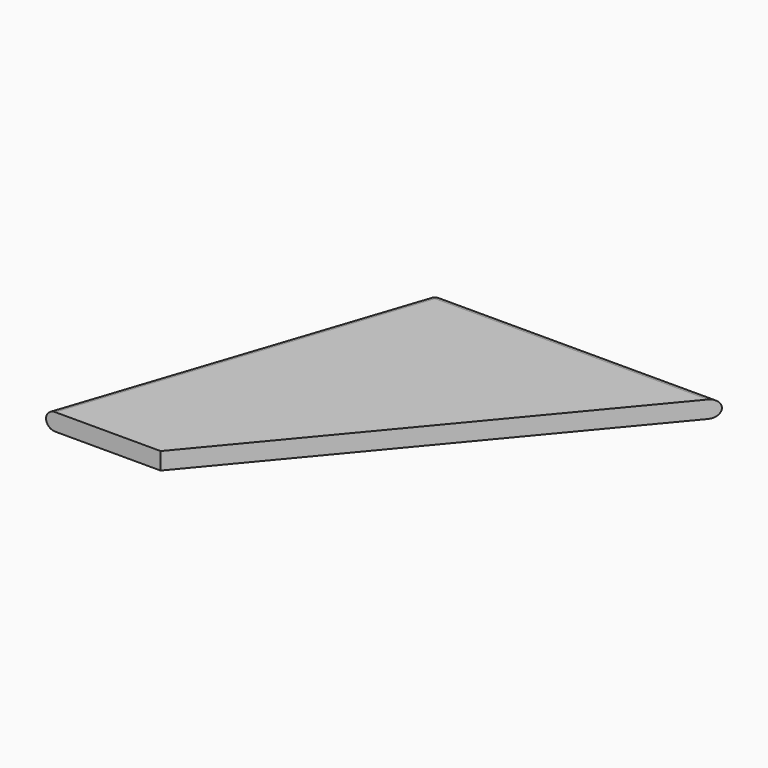
from build123d import *

# Parameters (mm, degrees)
F1_DEPTH = 3
F2_R     = 1.49999


# Not quite as in the source:
# - a fillet or chamfer is up to 0.001 mm smaller than in the source, because OpenCascade refuses the exact size


with BuildPart() as f1:
    # F0 (on Top) → F1 (new body)
    with BuildSketch(Plane.XY):
        Polygon((20, 60), (0, 0), (20, 0), (70, 60), align=None)
    extrude(amount=F1_DEPTH)

    # F2 (radius 1.5 in the source; OpenCascade refuses exactly that, so slightly less here)
    f2_edges = [f1.edges().sort_by_distance(p)[0] for p in [
        (45, 60, 3),
        (10, 30, 0),
        (10, 30, 3),
        (45, 60, 0),
        (20, 60, 1.5),
    ]]
    fillet(f2_edges, radius=F2_R)


solid = f1.part
